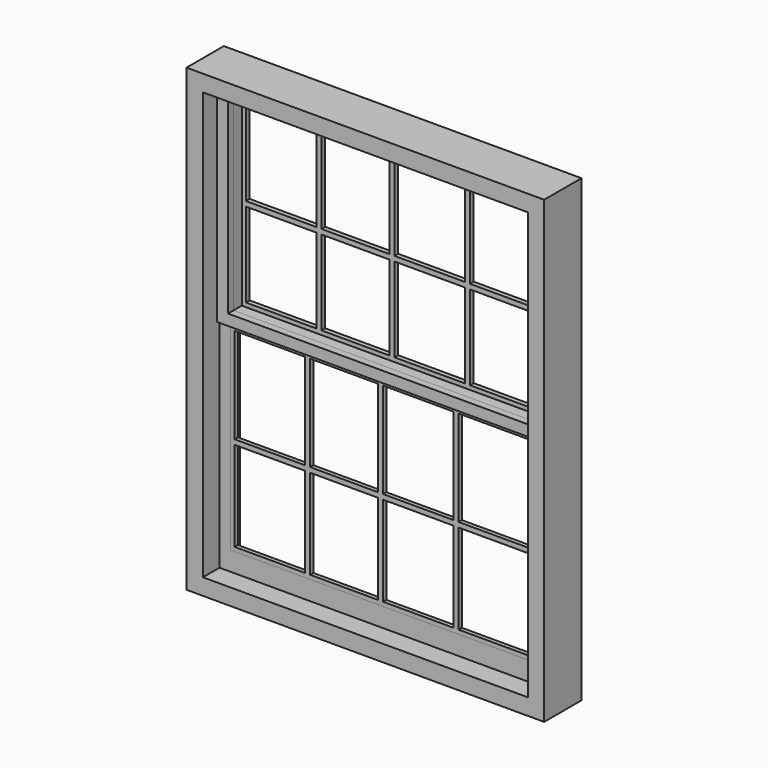
from build123d import *

# Parameters (mm, degrees)
F0_W          = 1310
F0_H          = 1684
F1_DEPTH      = 146
F1_DEPTH_BACK = 25
F0_W_2        = 1110
F0_H_2        = 687
F2_DEPTH      = 56
F3_START      = 1
F0_W_3        = 259
F0_H_3        = 309.25
F0_W_4        = 249
F0_H_4        = 329.75
F0_W_5        = 18
F3_DEPTH      = 17
F4_START      = 55
F0_H_5        = 727
F0_H_6        = 329.25
F0_H_7        = 349.75
F4_DEPTH      = 15
F5_SIZE2      = 12.670755226
F5_SIZE       = 80
F6_DEPTH      = 25
F8_DEPTH      = 16


# Not quite as in the source:
# - a feature names something its author has since deleted; it is built from what else it names


with BuildPart() as f1:
    # F0 (on Front) → F1 (new body, two sides)
    with BuildSketch(Plane.XZ) as f1_sk:
        with Locations((-655, 842)):
            Rectangle(F0_W, F0_H)
        Polygon((-1250, 1624), (-60, 1624), (-60, 857), (-60, 60), (-1250, 60), (-1250, 857), align=None, mode=Mode.SUBTRACT)
    extrude(amount=F1_DEPTH)
    extrude(f1_sk.sketch, amount=-F1_DEPTH_BACK)

    # F5
    f5_edges = [f1.edges().sort_by_distance(p)[0] for p in [
        (-655, 25, 60),
    ]]
    f5_side = f1.faces().sort_by_distance((-655, -60.5, 60))[0]
    chamfer(f5_edges, length=F5_SIZE, length2=F5_SIZE2, reference=f5_side)


with BuildPart() as f2:
    # F0 (on Front) → F2 (new body)
    with BuildSketch(Plane.XZ):
        Polygon((-60, 857), (-60, 1624), (-1250, 1624), (-1250, 857), (-1210, 857), (-100, 857), align=None)
        with Locations((-655, 1240.5)):
            Rectangle(F0_W_2, F0_H_2, mode=Mode.SUBTRACT)
    extrude(amount=F2_DEPTH)


with BuildPart() as f3:
    # F0 (on Front) → F3 (new body)
    with BuildSketch(Plane.XZ.offset(F3_START)):
        with Locations((-655, 1240.5)):
            Rectangle(F0_W_2, F0_H_2)
        with Locations((-1065.5, 1066.625)):
            Rectangle(F0_W_3, F0_H_3, mode=Mode.SUBTRACT)
        with Locations((-793.5, 1066.625)):
            Rectangle(F0_W_4, F0_H_3, mode=Mode.SUBTRACT)
        with Locations((-1065.5, 1404.125)):
            Rectangle(F0_W_3, F0_H_4, mode=Mode.SUBTRACT)
        with Locations((-793.5, 1404.125)):
            Rectangle(F0_W_4, F0_H_4, mode=Mode.SUBTRACT)
        Polygon((-374, 1221.25), (-115, 1221.25), (-115, 912), (-374, 912), (-392, 912), (-651, 912), (-651, 1221.25), (-392, 1221.25), align=None, mode=Mode.SUBTRACT)
        with Locations((-521.5, 1404.125)):
            Rectangle(F0_W_3, F0_H_4, mode=Mode.SUBTRACT)
        with Locations((-244.5, 1404.125)):
            Rectangle(F0_W_3, F0_H_4, mode=Mode.SUBTRACT)
        with Locations((-383, 1066.625)):
            Rectangle(F0_W_5, F0_H_3)
    extrude(amount=F3_DEPTH)


with BuildPart() as f4:
    # F0 (on Front) → F4 (new body)
    with BuildSketch(Plane.XZ.offset(F4_START)):
        with Locations((-655, 493.5)):
            Rectangle(F0_W_2, F0_H_5)
        with Locations((-1065.5, 309.625)):
            Rectangle(F0_W_3, F0_H_6, mode=Mode.SUBTRACT)
        with Locations((-793.5, 309.625)):
            Rectangle(F0_W_4, F0_H_6, mode=Mode.SUBTRACT)
        with Locations((-1065.5, 667.125)):
            Rectangle(F0_W_3, F0_H_7, mode=Mode.SUBTRACT)
        with Locations((-793.5, 667.125)):
            Rectangle(F0_W_4, F0_H_7, mode=Mode.SUBTRACT)
        Polygon((-651, 474.25), (-467.1856169297, 474.25), (-392, 474.25), (-392, 145), (-534.5, 145), (-651, 145), align=None, mode=Mode.SUBTRACT)
        with Locations((-244.5, 309.625)):
            Rectangle(F0_W_3, F0_H_6, mode=Mode.SUBTRACT)
        Polygon((-651, 842), (-392, 842), (-392, 492.25), (-463.5055595409, 492.25), (-651, 492.25), align=None, mode=Mode.SUBTRACT)
        with Locations((-244.5, 667.125)):
            Rectangle(F0_W_3, F0_H_7, mode=Mode.SUBTRACT)
    extrude(amount=F4_DEPTH)


with BuildPart() as f6:
    # F6 (new): a face of the model
    f6_faces = [f2.part.faces().sort_by_distance(p)[0] for p in [
        (-74.1576445781, -56, 1240.5),
    ]]
    extrude(f6_faces, amount=F6_DEPTH)


with BuildPart() as f8:
    # F7 (on face) → F8 (new body)
    with BuildSketch(Plane.XZ.offset(70)):
        Polygon((-1210, 857), (-1250.9673437476, 857), (-1250.9673437476, 60), (-60, 60), (-60, 857), (-100, 857), (-100, 130), (-1210, 130), align=None)
    extrude(amount=-F8_DEPTH)


solid = Compound([f1.part, f2.part, f3.part, f4.part, f6.part, f8.part])
